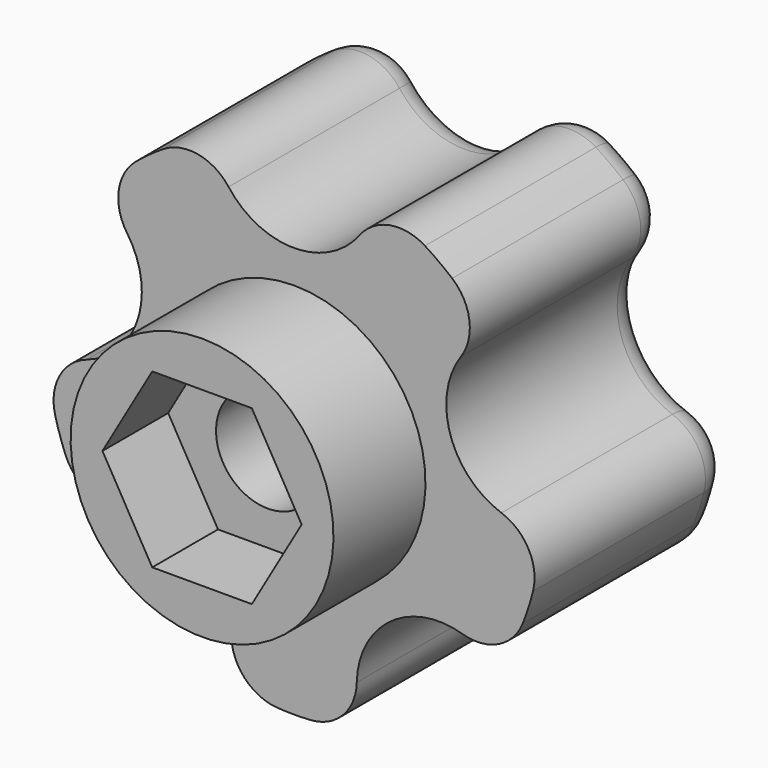
from build123d import *

# Parameters (mm, degrees)
F2_R        = 5
F3_DEPTH    = 15
F4_T1_DEPTH = 31.851779741
F6_DEPTH    = 5
F7_D        = 6.3
F8_R        = 2


# Not quite as in the source:
# - a fillet or chamfer that OpenCascade refuses, or shapes differently, is made with other operations: its cross-section is extruded or revolved along the edge and cut away or added


with BuildPart() as f1:
    # F0 (on Right) → F1 (revolve)
    with BuildSketch(Plane.YZ):
        Polygon((-22, 0), (0, 0), (0, 15), (-15, 15), (-15, 8), (-22, 8), align=None)
    revolve(axis=Axis((0, -11, 0), (0, -1, 0)))

    # F2 (on face) → F3 (cut)
    with BuildSketch(Plane(origin=(0, 0, 0), x_dir=(-1, 0, 0), z_dir=(0, 1, 0))):
        with Locations((0, 15)):
            Circle(F2_R)
        with Locations((-14.2658477444, 4.6352549156)):
            Circle(F2_R)
        with Locations((-8.8167787844, -12.1352549156)):
            Circle(F2_R)
        with Locations((8.8167787844, -12.1352549156)):
            Circle(F2_R)
        with Locations((14.2658477444, 4.6352549156)):
            Circle(F2_R)
    extrude(amount=-F3_DEPTH, mode=Mode.SUBTRACT)

    # F4: fillet of radius 3 on 10 edges, made by hand

    # F4_s2 → F4_t1 (cut)
    with BuildSketch(Plane.XZ.offset(-8.4258898705)):
        with BuildLine():
            ThreePointArc((14.5487698044, -3.6514787659), (14.2786844682, -1.4956481826), (12.6240778064, -0.0875187896))
            ThreePointArc((12.6240778064, -0.0875187896), (13.7969148622, -0.3427067106), (14.9967749751, -0.3110311036))
            ThreePointArc((14.9967749751, -0.3110311036), (14.8668911251, -1.993877698), (14.5487698044, -3.6514787659))
        make_face()
        with BuildLine():
            ThreePointArc((10.1616512299, 7.4910509465), (10.6725784478, 9.6028049498), (9.6239166514, 11.5056607062))
            ThreePointArc((9.6239166514, 11.5056607062), (10.855595668, 10.3516202931), (11.94982632, 9.0665126108))
            ThreePointArc((11.94982632, 9.0665126108), (10.9605006431, 8.3868786361), (10.1616512299, 7.4910509465))
        make_face()
        with BuildLine():
            ThreePointArc((1.0230544424, -14.9650713198), (2.9899102079, -14.0420166136), (3.8178192654, -12.0332562533))
            ThreePointArc((3.8178192654, -12.0332562533), (3.9375477121, -13.2275479821), (4.3384501703, -14.3588944602))
            ThreePointArc((4.3384501703, -14.3588944602), (2.6978316338, -14.755395775), (1.0230544424, -14.9650713198))
        make_face()
        with BuildLine():
            ThreePointArc((10.2645357375, -7.3494425703), (12.4308183364, -7.1827953553), (13.9164873867, -5.5974439539))
            ThreePointArc((13.9164873867, -5.5974439539), (13.1995394795, -7.1254584084), (12.3154653113, -8.5632537137))
            ThreePointArc((12.3154653113, -8.5632537137), (11.3633765438, -7.8323675302), (10.2645357375, -7.3494425703))
        make_face()
        with BuildLine():
            ThreePointArc((-13.9164873867, -5.5974439539), (-12.4308183364, -7.1827953553), (-10.2645357375, -7.3494425703))
            ThreePointArc((-10.2645357375, -7.3494425703), (-11.3633765438, -7.8323675302), (-12.3154653113, -8.5632537137))
            ThreePointArc((-12.3154653113, -8.5632537137), (-13.1995394795, -7.1254584084), (-13.9164873867, -5.5974439539))
        make_face()
        with BuildLine():
            ThreePointArc((-3.8178192654, -12.0332562533), (-2.9899102079, -14.0420166136), (-1.0230544424, -14.9650713198))
            ThreePointArc((-1.0230544424, -14.9650713198), (-2.6978316338, -14.755395775), (-4.3384501703, -14.3588944602))
            ThreePointArc((-4.3384501703, -14.3588944602), (-3.9375477121, -13.2275479821), (-3.8178192654, -12.0332562533))
        make_face()
        with BuildLine():
            ThreePointArc((-12.6240778064, -0.0875187896), (-14.2786844682, -1.4956481826), (-14.5487698044, -3.6514787659))
            ThreePointArc((-14.5487698044, -3.6514787659), (-14.8668911251, -1.993877698), (-14.9967749751, -0.3110311036))
            ThreePointArc((-14.9967749751, -0.3110311036), (-13.7969148622, -0.3427067106), (-12.6240778064, -0.0875187896))
        make_face()
        with BuildLine():
            ThreePointArc((-10.1616512299, 7.4910509465), (-10.6725784478, 9.6028049498), (-9.6239166514, 11.5056607062))
            ThreePointArc((-9.6239166514, 11.5056607062), (-10.855595668, 10.3516202931), (-11.94982632, 9.0665126108))
            ThreePointArc((-11.94982632, 9.0665126108), (-10.9605006431, 8.3868786361), (-10.1616512299, 7.4910509465))
        make_face()
        with BuildLine():
            ThreePointArc((7.9685797912, 12.7083333333), (5.8348021081, 13.1176552016), (3.9842898956, 11.9791666667))
            ThreePointArc((3.9842898956, 11.9791666667), (4.5894146126, 13.0157435868), (4.9300664859, 14.1666666667))
            ThreePointArc((4.9300664859, 14.1666666667), (6.4904123885, 13.5231115882), (7.9685797912, 12.7083333333))
        make_face()
        with BuildLine():
            ThreePointArc((-3.9842898956, 11.9791666667), (-5.8348021081, 13.1176552016), (-7.9685797912, 12.7083333333))
            ThreePointArc((-7.9685797912, 12.7083333333), (-6.4904123885, 13.5231115882), (-4.9300664859, 14.1666666667))
            ThreePointArc((-4.9300664859, 14.1666666667), (-4.5894146126, 13.0157435868), (-3.9842898956, 11.9791666667))
        make_face()
    extrude(amount=F4_T1_DEPTH, mode=Mode.SUBTRACT)

    # F5 (on face) → F6 (cut)
    with BuildSketch(Plane.XZ.offset(22)):
        Polygon((3.0310889132, 5.25), (-3.0310889132, 5.25), (-6.0621778265, 0), (-3.0310889132, -5.25), (3.0310889132, -5.25), (6.0621778265, 0), align=None)
    extrude(amount=-F6_DEPTH, mode=Mode.SUBTRACT)

    # F7 (through all)
    with Locations(Plane.XZ.offset(22)):
        with Locations((0, 0)):
            Hole(F7_D / 2)

    # F8
    f8_edges = [f1.edges().sort_by_distance(p)[0] for p in [
        (-8.816779, 0, 12.135255),
        (-5.834802, 0, 13.117655),
        (-10.672578, 0, 9.602805),
        (0, 0, 10),
        (-9.510565, 0, 3.09017),
        (5.834802, 0, 13.117655),
        (-14.278684, 0, -1.495648),
        (8.816779, 0, 12.135255),
        (-14.265848, 0, -4.635255),
        (10.672578, 0, 9.602805),
        (-12.430818, 0, -7.182795),
        (9.510565, 0, 3.09017),
        (-5.877853, 0, -8.09017),
        (14.278684, 0, -1.495648),
        (-2.98991, 0, -14.042017),
        (14.265848, 0, -4.635255),
        (0, 0, -15),
        (12.430818, 0, -7.182795),
        (2.98991, 0, -14.042017),
        (5.877853, 0, -8.09017),
    ]]
    fillet(f8_edges, radius=F8_R)


solid = f1.part
